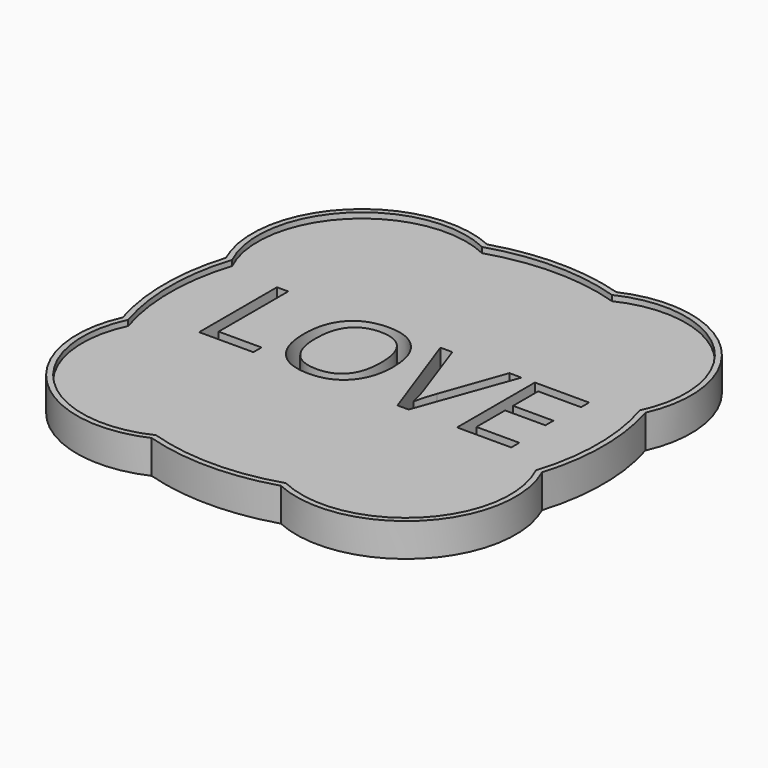
from build123d import *

# Parameters (mm, degrees)
F1_DEPTH     = 25.4
F2_TEXT_SIZE = 124.2101241643
F3_DEPTH     = 25.4
F5_DEPTH     = 5


# Not quite as in the source:
# - Text() gives the source's letters only with a copy of the font that has no kerning and outlines rounded to 1/6400 em; it was checked with that copy


with BuildPart() as f1:
    # F0 (on Top) → F1 (new body)
    with BuildSketch(Plane.XY):
        with BuildLine():
            ThreePointArc((-58.8562172234, 191.1437827766), (-170.7106781187, 170.7106781187), (-191.1437827766, 58.8562172234))
            ThreePointArc((-191.1437827766, 58.8562172234), (-200, 0), (-191.1437827766, -58.8562172234))
            ThreePointArc((-191.1437827766, -58.8562172234), (-170.7106781187, -170.7106781187), (-58.8562172234, -191.1437827766))
            ThreePointArc((-58.8562172234, -191.1437827766), (0, -200), (58.8562172234, -191.1437827766))
            ThreePointArc((58.8562172234, -191.1437827766), (170.7106781187, -170.7106781187), (191.1437827766, -58.8562172234))
            ThreePointArc((191.1437827766, -58.8562172234), (200, 0), (191.1437827766, 58.8562172234))
            ThreePointArc((191.1437827766, 58.8562172234), (170.7106781187, 170.7106781187), (58.8562172234, 191.1437827766))
            ThreePointArc((58.8562172234, 191.1437827766), (0, 200), (-58.8562172234, 191.1437827766))
        make_face()
    extrude(amount=F1_DEPTH)

    # F2 (on face) → F3 (cut)
    with BuildSketch(Plane.XY.offset(25.4)):
        with Locations((-152.6364424653, -35.1024734998)):
            Text('LOVE', F2_TEXT_SIZE, font='Open Sans', text_align=(TextAlign.LEFT, TextAlign.BOTTOM))
    extrude(amount=-F3_DEPTH, mode=Mode.SUBTRACT)

    # F4 (on face) → F5 (join)
    with BuildSketch(Plane.XY.offset(25.4)):
        with BuildLine():
            ThreePointArc((58.8562172234, 191.1437827766), (0, 200), (-58.8562172234, 191.1437827766))
            ThreePointArc((-58.8562172234, 191.1437827766), (-170.7106781187, 170.7106781187), (-191.1437827766, 58.8562172234))
            ThreePointArc((-191.1437827766, 58.8562172234), (-200, 0), (-191.1437827766, -58.8562172234))
            ThreePointArc((-191.1437827766, -58.8562172234), (-170.7106781187, -170.7106781187), (-58.8562172234, -191.1437827766))
            ThreePointArc((-58.8562172234, -191.1437827766), (0, -200), (58.8562172234, -191.1437827766))
            ThreePointArc((58.8562172234, -191.1437827766), (170.7106781187, -170.7106781187), (191.1437827766, -58.8562172234))
            ThreePointArc((191.1437827766, -58.8562172234), (200, 0), (191.1437827766, 58.8562172234))
            ThreePointArc((191.1437827766, 58.8562172234), (170.7106781187, 170.7106781187), (58.8562172234, 191.1437827766))
        make_face()
        with BuildLine():
            ThreePointArc((59.2050554941, -185.7949445059), (0, -195), (-59.2050554941, -185.7949445059))
            ThreePointArc((-59.2050554941, -185.7949445059), (-167.1751442127, -167.1751442127), (-185.7949445059, -59.2050554941))
            ThreePointArc((-185.7949445059, -59.2050554941), (-195, 0), (-185.7949445059, 59.2050554941))
            ThreePointArc((-185.7949445059, 59.2050554941), (-167.1751442127, 167.1751442127), (-59.2050554941, 185.7949445059))
            ThreePointArc((-59.2050554941, 185.7949445059), (0, 195), (59.2050554941, 185.7949445059))
            ThreePointArc((59.2050554941, 185.7949445059), (167.1751442127, 167.1751442127), (185.7949445059, 59.2050554941))
            ThreePointArc((185.7949445059, 59.2050554941), (195, 0), (185.7949445059, -59.2050554941))
            ThreePointArc((185.7949445059, -59.2050554941), (167.1751442127, -167.1751442127), (59.2050554941, -185.7949445059))
        make_face(mode=Mode.SUBTRACT)
    extrude(amount=F5_DEPTH)


solid = f1.part
